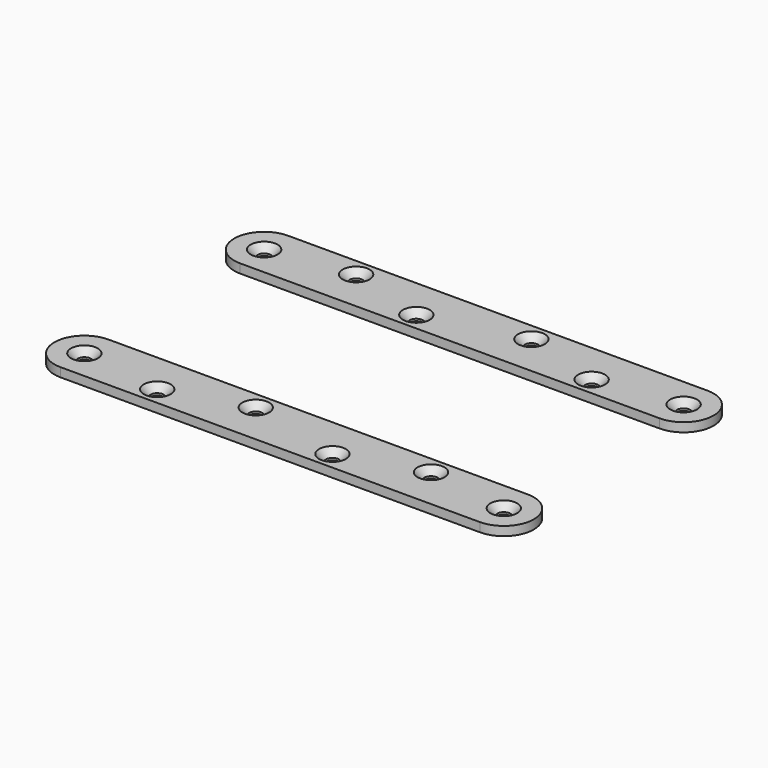
from build123d import *

# Parameters (mm, degrees)
F1_DEPTH       = 3
F2_D           = 4.4
F2_CSINK_D     = 8.96
F2_CSINK_ANGLE = 90


# Not quite as in the source:
# - a feature names something its author has since deleted; it is built from what else it names


with BuildPart() as f1:
    # F0 (on Top) → F1 (new body)
    with BuildSketch(Plane.XY):
        with BuildLine():
            ThreePointArc((70, 27.5), (80, 37.5), (70, 47.5))
            Line((70, 47.5), (-70, 47.5))
            ThreePointArc((-70, 47.5), (-80, 37.5), (-70, 27.5))
            Line((-70, 27.5), (70, 27.5))
        make_face()
    extrude(amount=-F1_DEPTH)

    # F2 (through all)
    with Locations(Plane.XY):
        with Locations((-70, 37.5), (-42.5, 41.5), (-16, 33.5), (16, 41.5), (42.5, 33.5), (70, 37.5)):
            CounterSinkHole(F2_D / 2, F2_CSINK_D / 2, counter_sink_angle=F2_CSINK_ANGLE)


with BuildPart() as f3_1:
    # F3: instance of F1
    add(f1.part.mirror(Plane.XZ))


solid = Compound([f1.part, f3_1.part])
